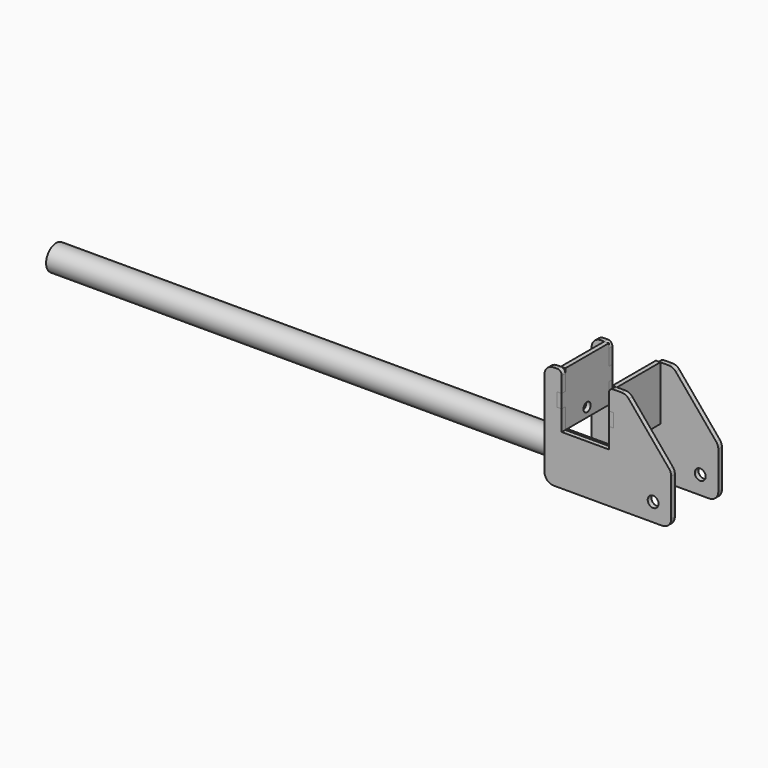
from build123d import *

# Parameters (mm, degrees)
F0_R         = 6
F1_DEPTH     = 5
F2_W         = 5
F2_H         = 15
F3_DEPTH     = 5
F4_R         = 5
F5_DEPTH     = 25
F7_W         = 75
F7_H         = 70
F7_R         = 26
F8_DEPTH     = 40
F9_W         = 70
F9_H         = 30
F10_DEPTH    = 70
F11_T1_DEPTH = 115
F12_R        = 5
F13_R        = 14
F14_DEPTH    = 25
F15_R        = 14
F15_R_2      = 10
F16_DEPTH    = 650
F17_R        = 2.5
F18_DEPTH    = 60


# Not quite as in the source:
# - a fillet or chamfer that OpenCascade refuses, or shapes differently, is made with other operations: its cross-section is extruded or revolved along the edge and cut away or added


with BuildPart() as f1:
    # F0 (on Front) → F1 (new body)
    with BuildSketch(Plane.XZ):
        with BuildLine():
            ThreePointArc((0, 10), (2.9289321881, 2.9289321881), (10, 0))
            Line((10, 0), (130, 0))
            ThreePointArc((130, 0), (137.0710678119, 2.9289321881), (140, 10))
            Line((140, 10), (140, 51.3795006482))
            ThreePointArc((140, 51.3795006482), (139.4027157768, 54.7837532857), (137.682212796, 57.7813446448))
            Line((137.682212796, 57.7813446448), (92.9984633361, 111.4018439966))
            ThreePointArc((92.9984633361, 111.4018439966), (89.5578045027, 114.0558942122), (85.3162505402, 115))
            Line((85.3162505402, 115), (76, 115))
            ThreePointArc((76, 115), (72.4644660941, 113.5355339059), (71, 110))
            Line((71, 110), (71, 92.5))
            Line((71, 92.5), (76, 92.5))
            Line((76, 92.5), (76, 77.5))
            Line((76, 77.5), (71, 77.5))
            Line((71, 77.5), (71, 55))
            Line((71, 55), (19, 55))
            Line((19, 55), (19, 77.5))
            Line((19, 77.5), (14, 77.5))
            Line((14, 77.5), (14, 92.5))
            Line((14, 92.5), (19, 92.5))
            Line((19, 92.5), (19, 110))
            ThreePointArc((19, 110), (17.5355339059, 113.5355339059), (14, 115))
            Line((14, 115), (10, 115))
            ThreePointArc((10, 115), (2.9289321881, 112.0710678119), (0, 105))
            Line((0, 105), (0, 10))
        make_face()
        with Locations((120, 20)):
            Circle(F0_R, mode=Mode.SUBTRACT)
    extrude(amount=F1_DEPTH)


with BuildPart() as f3:
    # F2 (on face) → F3 (new body)
    with BuildSketch(Plane(origin=(76, 0, 0), x_dir=(0, -1, 0), z_dir=(-1, 0, 0))):
        Polygon((5, 77.5), (5, 92.5), (0, 92.5), (0, 115), (-60, 115), (-60, 92.5), (-60, 77.5), (-60, 55), (0, 55), (0, 77.5), align=None)
        with Locations((-62.5, 85)):
            Rectangle(F2_W, F2_H)
    extrude(amount=F3_DEPTH)

    # F4 (on face) → F5 (cut)
    with BuildSketch(Plane.YZ.offset(76)):
        with Locations((30, 65)):
            Circle(F4_R)
    extrude(amount=-F5_DEPTH, mode=Mode.SUBTRACT)


with BuildPart() as f8:
    # F7 (on offset) → F8 (new body)
    with BuildSketch(Plane(origin=(0, 10, 0), x_dir=(-1, 0, 0), z_dir=(0, 1, 0))):
        with Locations((-120, 20)):
            Rectangle(F7_W, F7_H)
        with Locations((-120, 20)):
            Circle(F7_R, mode=Mode.SUBTRACT)
    extrude(amount=F8_DEPTH)

    # F9 (on face) → F10 (cut)
    with BuildSketch(Plane.XY.offset(55)):
        with Locations((122.5, 30)):
            Rectangle(F9_W, F9_H)
    extrude(amount=-F10_DEPTH, mode=Mode.SUBTRACT)

    # F11: fillet of radius 15 on 2 edges, made by hand

    # F11_s2 → F11_t1 (cut)
    with BuildSketch(Plane.XZ.offset(-87.5)):
        with BuildLine():
            ThreePointArc((82.5, 0), (86.8933982822, -10.6066017178), (97.5, -15))
            Line((97.5, -15), (82.5, -15))
            Line((82.5, -15), (82.5, 0))
        make_face()
        with BuildLine():
            ThreePointArc((82.5, 40), (86.8933982822, 50.6066017178), (97.5, 55))
            Line((97.5, 55), (82.5, 55))
            Line((82.5, 55), (82.5, 40))
        make_face()
    extrude(amount=F11_T1_DEPTH, mode=Mode.SUBTRACT)

    # F12
    f12_edges = [f8.edges().sort_by_distance(p)[0] for p in [
        (157.5, 47.5, 55),
        (157.5, 12.5, 55),
        (157.5, 47.5, -15),
        (157.5, 12.5, -15),
    ]]
    fillet(f12_edges, radius=F12_R)

    # F13 (on face) → F14 (cut)
    with BuildSketch(Plane(origin=(82.5, 0, 0), x_dir=(0, -1, 0), z_dir=(-1, 0, 0))):
        with Locations((-30, 20)):
            Circle(F13_R)
    extrude(amount=-F14_DEPTH, mode=Mode.SUBTRACT)


with BuildPart() as f16:
    # F15 (on face) → F16 (new body)
    with BuildSketch(Plane(origin=(82.5, 0, 0), x_dir=(0, -1, 0), z_dir=(-1, 0, 0))):
        with Locations((-30, 20)):
            Circle(F15_R)
        with Locations((-30, 20)):
            Circle(F15_R_2, mode=Mode.SUBTRACT)
    extrude(amount=F16_DEPTH)


with BuildPart() as f18:
    # F17 (on face) → F18 (new body)
    with BuildSketch(Plane(origin=(0, 0, 0), x_dir=(-1, 0, 0), z_dir=(0, 1, 0))):
        with Locations((-120, 20)):
            Circle(F17_R)
    extrude(amount=F18_DEPTH)


with BuildPart() as f21_1:
    # F21: copy of F1
    add(f1.part.moved(Location((0, 65, 0))))


with BuildPart() as f22_1:
    # F22: copy of F3
    add(f3.part.moved(Location((-57, 0, 0))))


solid = Compound([f1.part, f3.part, f16.part, f21_1.part, f22_1.part])
